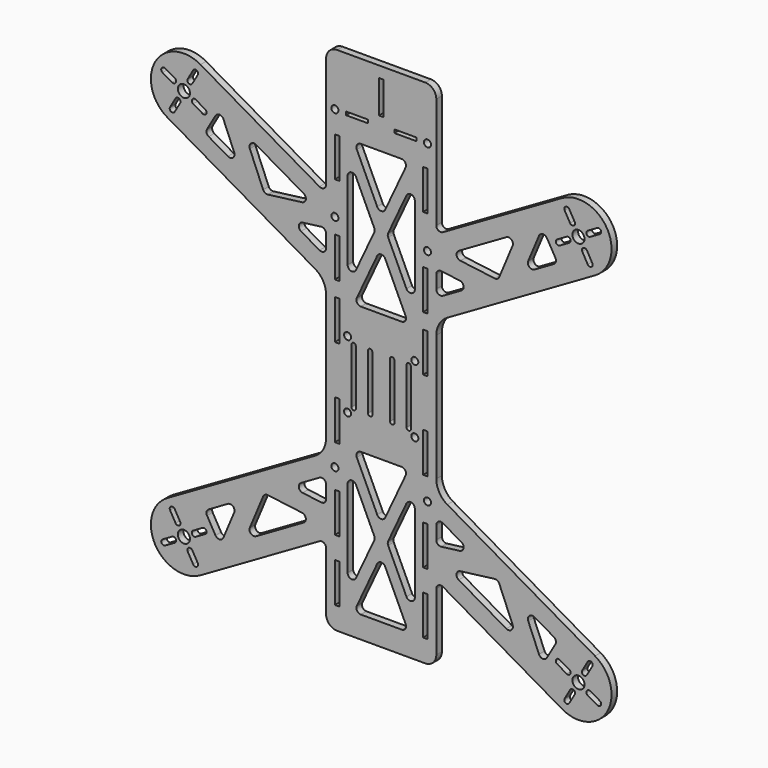
from build123d import *

# Parameters (mm, degrees)
F0_R     = 2.75
F0_W     = 2
F0_H     = 18
F0_R_2   = 1.6
F0_W_2   = 10
F0_H_2   = 1.5
F0_H_3   = 15
F1_DEPTH = 3.175


# Not quite as in the source:
# - ends of sketch curves that miss each other by under 0.0002 mm in the source are joined


with BuildPart() as f1:
    # F0 (on Front) → F1 (new body)
    with BuildSketch(Plane.XZ):
        with BuildLine():
            ThreePointArc((-25, 60.545517), (-26.0000001748, 58.8134660915), (-28.0000003497, 58.8134663943))
            Line((-28.0000003497, 58.8134663943), (-82, 89.990381))
            ThreePointArc((-82, 89.990381), (-102.4903810426, 84.5000000246), (-97.0000000246, 64.0096189574))
            Line((-97.0000000246, 64.0096189574), (-30, 25.327151))
            ThreePointArc((-30, 25.327151), (-26.3397459574, 21.6668969918), (-25, 16.666897))
            Line((-25, 16.666897), (-25, -40.666897))
            ThreePointArc((-25, -40.666897), (-26.3397459574, -45.6668969918), (-29.9999999836, -49.3271510284))
            Line((-29.9999999836, -49.3271510284), (-97, -88.009619))
            ThreePointArc((-97, -88.009619), (-102.4903810426, -108.5000000246), (-81.9999999754, -113.9903810426))
            Line((-81.9999999754, -113.9903810426), (-28, -82.813467))
            ThreePointArc((-28, -82.813467), (-26.0000001748, -82.8134660915), (-25, -84.545517))
            Line((-25, -84.545517), (-25, -111))
            ThreePointArc((-25, -111), (-23.5355339059, -114.5355339059), (-20, -116))
            Line((-20, -116), (20, -116))
            ThreePointArc((20, -116), (23.5355339059, -114.5355339059), (25, -111))
            Line((25, -111), (25, -84.545517))
            ThreePointArc((25, -84.545517), (26.0000001748, -82.8134660915), (28.0000003497, -82.8134663943))
            Line((28.0000003497, -82.8134663943), (82, -113.990381))
            ThreePointArc((82, -113.990381), (102.4903810426, -108.5000000246), (97.0000000246, -88.0096189574))
            Line((97.0000000246, -88.0096189574), (30, -49.327151))
            ThreePointArc((30, -49.327151), (26.3397459574, -45.6668969918), (25, -40.666897))
            Line((25, -40.666897), (25, 16.666897))
            ThreePointArc((25, 16.666897), (26.3397459574, 21.6668969918), (29.9999999836, 25.3271510284))
            Line((29.9999999836, 25.3271510284), (97, 64.009619))
            ThreePointArc((97, 64.009619), (102.4903810426, 84.5000000246), (81.9999999754, 89.9903810426))
            Line((81.9999999754, 89.9903810426), (28, 58.813467))
            ThreePointArc((28, 58.813467), (26.0000001748, 58.8134660915), (25, 60.545517))
            Line((25, 60.545517), (25, 111))
            ThreePointArc((25, 111), (23.5355339059, 114.5355339059), (20, 116))
            Line((20, 116), (-20, 116))
            ThreePointArc((-20, 116), (-23.5355339059, 114.5355339059), (-25, 111))
            Line((-25, 111), (-25, 60.545517))
        make_face()
        with BuildLine():
            ThreePointArc((-94.8631402098, -102.7107696366), (-93.2239096366, -103.1499997902), (-93.6631397902, -104.7892303634))
            Line((-93.6631397902, -104.7892303634), (-97.993267, -107.28923))
            ThreePointArc((-97.993267, -107.28923), (-99.6324973634, -106.8500002098), (-99.1932672098, -105.2107696366))
            Line((-99.1932672098, -105.2107696366), (-94.8631402098, -102.7107696366))
        make_face(mode=Mode.SUBTRACT)
        with BuildLine():
            ThreePointArc((-87.7892303634, -106.3631402098), (-87.3500002098, -104.7239096366), (-85.7107696366, -105.1631397902))
            Line((-85.7107696366, -105.1631397902), (-83.21077, -109.493267))
            ThreePointArc((-83.21077, -109.493267), (-83.6499997902, -111.1324973634), (-85.2892303634, -110.6932672098))
            Line((-85.2892303634, -110.6932672098), (-87.7892303634, -106.3631402098))
        make_face(mode=Mode.SUBTRACT)
        with BuildLine():
            ThreePointArc((-91.2107696366, -95.6368597902), (-91.6499997902, -97.2760903634), (-93.2892303634, -96.8368602098))
            Line((-93.2892303634, -96.8368602098), (-95.78923, -92.506733))
            ThreePointArc((-95.78923, -92.506733), (-95.3500002098, -90.8675026366), (-93.7107696366, -91.3067327902))
            Line((-93.7107696366, -91.3067327902), (-91.2107696366, -95.6368597902))
        make_face(mode=Mode.SUBTRACT)
        with Locations((-89.5, -101)):
            Circle(F0_R, mode=Mode.SUBTRACT)
        with BuildLine():
            ThreePointArc((-84.1368597902, -99.2892303634), (-85.7760903634, -98.8500002098), (-85.3368602098, -97.2107696366))
            Line((-85.3368602098, -97.2107696366), (-81.006733, -94.71077))
            ThreePointArc((-81.006733, -94.71077), (-79.3675026366, -95.1499997902), (-79.8067327902, -96.7892303634))
            Line((-79.8067327902, -96.7892303634), (-84.1368597902, -99.2892303634))
        make_face(mode=Mode.SUBTRACT)
        with BuildLine():
            ThreePointArc((-79.0096188557, -89.1698729167), (-79.2094196277, -87.6522348169), (-78.2775679167, -86.4378221443))
            Line((-78.2775679167, -86.4378221443), (-69.539197, -81.392721))
            ThreePointArc((-69.539197, -81.392721), (-67.2175903894, -81.6236537612), (-66.6944217571, -83.8973031017))
            Line((-66.6944217571, -83.8973031017), (-71.592563, -95.593878))
            ThreePointArc((-71.592563, -95.593878), (-73.3104041105, -96.8173148824), (-75.1693888557, -95.8213469167))
            Line((-75.1693888557, -95.8213469167), (-79.0096188557, -89.1698729167))
        make_face(mode=Mode.SUBTRACT)
        with Locations((-20, -97)):
            Rectangle(F0_W, F0_H, mode=Mode.SUBTRACT)
        with BuildLine():
            ThreePointArc((-9.257183, -106), (-10.9439659593, -105.0745991105), (-11.0697984676, -103.1547632482))
            Line((-11.0697984676, -103.1547632482), (-1.812616, -83.302671))
            ThreePointArc((-1.812616, -83.302671), (0, -82.147907), (1.8126158507, -83.3026710696))
            Line((1.8126158507, -83.3026710696), (11.069799, -103.154763))
            ThreePointArc((11.069799, -103.154763), (10.9439659593, -105.0745991105), (9.257183, -106))
            Line((9.257183, -106), (-9.257183, -106))
        make_face(mode=Mode.SUBTRACT)
        with BuildLine():
            ThreePointArc((-56.7584760833, -90.1795758557), (-59.0800826106, -89.9486432388), (-59.6032512429, -87.6749938983))
            Line((-59.6032512429, -87.6749938983), (-53.553313, -73.227971))
            ThreePointArc((-53.553313, -73.227971), (-52.708538039, -72.268451215), (-51.4551820272, -72.0166142131))
            Line((-51.4551820272, -72.0166142131), (-35.918724, -74.000726))
            ThreePointArc((-35.918724, -74.000726), (-34.2112701558, -75.5906282709), (-35.1720800833, -77.7166648557))
            Line((-35.1720800833, -77.7166648557), (-56.7584760833, -90.1795758557))
        make_face(mode=Mode.SUBTRACT)
        with BuildLine():
            ThreePointArc((-35.6447150984, -65.9707467709), (-37.3521688567, -64.380844667), (-36.3913589167, -62.2548081443))
            Line((-36.3913589167, -62.2548081443), (-28, -57.410055))
            ThreePointArc((-28, -57.410055), (-26.0000001748, -57.4100540915), (-25, -59.142105))
            Line((-25, -59.142105), (-25, -65.058492))
            ThreePointArc((-25, -65.058492), (-25.6783933917, -66.5596102408), (-27.2533559728, -67.0423797869))
            Line((-27.2533559728, -67.0423797869), (-35.6447150984, -65.9707467709))
        make_face(mode=Mode.SUBTRACT)
        with BuildLine():
            ThreePointArc((-11.4373841493, -92.1120459304), (-13.6828789084, -93.2194020851), (-15.25, -91.26681))
            Line((-15.25, -91.26681), (-15.25, -55.73319))
            ThreePointArc((-15.25, -55.73319), (-13.6828789084, -53.7805979149), (-11.4373841493, -54.8879540696))
            Line((-11.4373841493, -54.8879540696), (-3.152585, -72.654763))
            ThreePointArc((-3.152585, -72.654763), (-2.965201, -73.5), (-3.1525855324, -74.3452367518))
            Line((-3.1525855324, -74.3452367518), (-11.4373841493, -92.1120459304))
        make_face(mode=Mode.SUBTRACT)
        with Locations((-20, -69)):
            Rectangle(F0_W, F0_H, mode=Mode.SUBTRACT)
        with Locations((-21, -51)):
            Circle(F0_R_2, mode=Mode.SUBTRACT)
        with BuildLine():
            ThreePointArc((1.8126158507, -63.6973289304), (0, -64.852093), (-1.8126158507, -63.6973289304))
            Line((-1.8126158507, -63.6973289304), (-11.069799, -43.845237))
            ThreePointArc((-11.069799, -43.845237), (-10.9439659593, -41.9254008895), (-9.257183, -41))
            Line((-9.257183, -41), (9.257183, -41))
            ThreePointArc((9.257183, -41), (10.9439659593, -41.9254008895), (11.0697984676, -43.8452367518))
            Line((11.0697984676, -43.8452367518), (1.8126158507, -63.6973289304))
        make_face(mode=Mode.SUBTRACT)
        with Locations((-20, -32)):
            Rectangle(F0_W, F0_H, mode=Mode.SUBTRACT)
        with Locations((-15.25, -27.25)):
            Circle(F0_R_2, mode=Mode.SUBTRACT)
        with BuildLine():
            Line((-13.5, -24.5), (-13.5, 0.5))
            ThreePointArc((-13.5, 0.5), (-12.5, 1.5), (-11.5, 0.5))
            Line((-11.5, 0.5), (-11.5, -24.5))
            ThreePointArc((-11.5, -24.5), (-12.5, -25.5), (-13.5, -24.5))
        make_face(mode=Mode.SUBTRACT)
        with BuildLine():
            Line((-6, -24.5), (-6, 0.5))
            ThreePointArc((-6, 0.5), (-5, 1.5), (-4, 0.5))
            Line((-4, 0.5), (-4, -24.5))
            ThreePointArc((-4, -24.5), (-5, -25.5), (-6, -24.5))
        make_face(mode=Mode.SUBTRACT)
        with Locations((20, -97)):
            Rectangle(F0_W, F0_H, mode=Mode.SUBTRACT)
        with BuildLine():
            ThreePointArc((15.25, -91.26681), (13.6828789084, -93.2194020851), (11.4373841493, -92.1120459304))
            Line((11.4373841493, -92.1120459304), (3.152585, -74.345237))
            ThreePointArc((3.152585, -74.345237), (2.965201, -73.5), (3.1525855324, -72.6547632482))
            Line((3.1525855324, -72.6547632482), (11.437384, -54.887954))
            ThreePointArc((11.437384, -54.887954), (13.6828789084, -53.7805979149), (15.25, -55.73319))
            Line((15.25, -55.73319), (15.25, -91.26681))
        make_face(mode=Mode.SUBTRACT)
        with Locations((20, -69)):
            Rectangle(F0_W, F0_H, mode=Mode.SUBTRACT)
        with BuildLine():
            ThreePointArc((59.6032512429, -87.6749938983), (59.0800826106, -89.9486432388), (56.7584760833, -90.1795758557))
            Line((56.7584760833, -90.1795758557), (35.17208, -77.716665))
            ThreePointArc((35.17208, -77.716665), (34.2112701558, -75.5906282709), (35.9187240272, -74.0007262131))
            Line((35.9187240272, -74.0007262131), (51.455182, -72.016614))
            ThreePointArc((51.455182, -72.016614), (52.708538039, -72.268451215), (53.5533132429, -73.2279708983))
            Line((53.5533132429, -73.2279708983), (59.6032512429, -87.6749938983))
        make_face(mode=Mode.SUBTRACT)
        with BuildLine():
            ThreePointArc((36.3913589167, -62.2548081443), (37.3521688567, -64.380844667), (35.6447150984, -65.9707467709))
            Line((35.6447150984, -65.9707467709), (27.253356, -67.04238))
            ThreePointArc((27.253356, -67.04238), (25.6783933917, -66.5596102408), (25, -65.058492))
            Line((25, -65.058492), (25, -59.142105))
            ThreePointArc((25, -59.142105), (26.0000001748, -57.4100540915), (28.0000003497, -57.4100543943))
            Line((28.0000003497, -57.4100543943), (36.3913589167, -62.2548081443))
        make_face(mode=Mode.SUBTRACT)
        with BuildLine():
            ThreePointArc((78.2775679167, -86.4378221443), (79.2094196277, -87.6522348169), (79.0096188557, -89.1698729167))
            Line((79.0096188557, -89.1698729167), (75.169389, -95.821347))
            ThreePointArc((75.169389, -95.821347), (73.3104041105, -96.8173148824), (71.5925627571, -95.5938781017))
            Line((71.5925627571, -95.5938781017), (66.694422, -83.897303))
            ThreePointArc((66.694422, -83.897303), (67.2175903894, -81.6236537612), (69.5391969167, -81.3927211443))
            Line((69.5391969167, -81.3927211443), (78.2775679167, -86.4378221443))
        make_face(mode=Mode.SUBTRACT)
        with BuildLine():
            Line((83.21077, -109.493267), (85.71077, -105.16314))
            ThreePointArc((85.71077, -105.16314), (87.3500002098, -104.7239096366), (87.7892303634, -106.3631402098))
            Line((87.7892303634, -106.3631402098), (85.28923, -110.693267))
            ThreePointArc((85.28923, -110.693267), (83.6499997902, -111.1324973634), (83.21077, -109.493267))
        make_face(mode=Mode.SUBTRACT)
        with BuildLine():
            Line((97.993267, -107.28923), (93.66314, -104.78923))
            ThreePointArc((93.66314, -104.78923), (93.2239096366, -103.1499997902), (94.8631402098, -102.7107696366))
            Line((94.8631402098, -102.7107696366), (99.193267, -105.21077))
            ThreePointArc((99.193267, -105.21077), (99.6324973634, -106.8500002098), (97.993267, -107.28923))
        make_face(mode=Mode.SUBTRACT)
        with BuildLine():
            Line((81.006733, -94.71077), (85.33686, -97.21077))
            ThreePointArc((85.33686, -97.21077), (85.7760903634, -98.8500002098), (84.1368597902, -99.2892303634))
            Line((84.1368597902, -99.2892303634), (79.806733, -96.78923))
            ThreePointArc((79.806733, -96.78923), (79.3675026366, -95.1499997902), (81.006733, -94.71077))
        make_face(mode=Mode.SUBTRACT)
        with Locations((89.5, -101)):
            Circle(F0_R, mode=Mode.SUBTRACT)
        with BuildLine():
            Line((95.78923, -92.506733), (93.28923, -96.83686))
            ThreePointArc((93.28923, -96.83686), (91.6499997902, -97.2760903634), (91.2107696366, -95.6368597902))
            Line((91.2107696366, -95.6368597902), (93.71077, -91.306733))
            ThreePointArc((93.71077, -91.306733), (95.3500002098, -90.8675026366), (95.78923, -92.506733))
        make_face(mode=Mode.SUBTRACT)
        with Locations((21, -51)):
            Circle(F0_R_2, mode=Mode.SUBTRACT)
        with Locations((20, -32)):
            Rectangle(F0_W, F0_H, mode=Mode.SUBTRACT)
        with Locations((15.25, -27.25)):
            Circle(F0_R_2, mode=Mode.SUBTRACT)
        with BuildLine():
            ThreePointArc((4, 0.5), (5, 1.5), (6, 0.5))
            Line((6, 0.5), (6, -24.5))
            ThreePointArc((6, -24.5), (5, -25.5), (4, -24.5))
            Line((4, -24.5), (4, 0.5))
        make_face(mode=Mode.SUBTRACT)
        with BuildLine():
            ThreePointArc((11.5, 0.5), (12.5, 1.5), (13.5, 0.5))
            Line((13.5, 0.5), (13.5, -24.5))
            ThreePointArc((13.5, -24.5), (12.5, -25.5), (11.5, -24.5))
            Line((11.5, -24.5), (11.5, 0.5))
        make_face(mode=Mode.SUBTRACT)
        with Locations((-15.25, 3.25)):
            Circle(F0_R_2, mode=Mode.SUBTRACT)
        with Locations((-20, 8)):
            Rectangle(F0_W, F0_H, mode=Mode.SUBTRACT)
        with BuildLine():
            ThreePointArc((-9.257183, 17), (-10.9439659593, 17.9254008895), (-11.0697984676, 19.8452367518))
            Line((-11.0697984676, 19.8452367518), (-1.812616, 39.697329))
            ThreePointArc((-1.812616, 39.697329), (0, 40.852093), (1.8126158507, 39.6973289304))
            Line((1.8126158507, 39.6973289304), (11.069799, 19.845237))
            ThreePointArc((11.069799, 19.845237), (10.9439659593, 17.9254008895), (9.257183, 17))
            Line((9.257183, 17), (-9.257183, 17))
        make_face(mode=Mode.SUBTRACT)
        with BuildLine():
            ThreePointArc((-27.2533559728, 43.0423797869), (-25.6783933917, 42.5596102408), (-25, 41.058492))
            Line((-25, 41.058492), (-25, 35.142105))
            ThreePointArc((-25, 35.142105), (-26.0000001748, 33.4100540915), (-28.0000003497, 33.4100543943))
            Line((-28.0000003497, 33.4100543943), (-36.391359, 38.254808))
            ThreePointArc((-36.391359, 38.254808), (-37.3521688567, 40.380844667), (-35.6447150984, 41.9707467709))
            Line((-35.6447150984, 41.9707467709), (-27.2533559728, 43.0423797869))
        make_face(mode=Mode.SUBTRACT)
        with BuildLine():
            ThreePointArc((-35.1720800833, 53.7166648557), (-34.2112701558, 51.5906282709), (-35.9187240272, 50.0007262131))
            Line((-35.9187240272, 50.0007262131), (-51.455182, 48.016614))
            ThreePointArc((-51.455182, 48.016614), (-52.708538039, 48.268451215), (-53.5533132429, 49.2279708983))
            Line((-53.5533132429, 49.2279708983), (-59.603251, 63.674994))
            ThreePointArc((-59.603251, 63.674994), (-59.0800826106, 65.9486432388), (-56.7584760833, 66.1795758557))
            Line((-56.7584760833, 66.1795758557), (-35.1720800833, 53.7166648557))
        make_face(mode=Mode.SUBTRACT)
        with Locations((-20, 33)):
            Rectangle(F0_W, F0_H, mode=Mode.SUBTRACT)
        with Locations((-21, 49)):
            Circle(F0_R_2, mode=Mode.SUBTRACT)
        with BuildLine():
            ThreePointArc((-15.25, 67.26681), (-13.6828789084, 69.2194020851), (-11.4373841493, 68.1120459304))
            Line((-11.4373841493, 68.1120459304), (-3.152585, 50.345237))
            ThreePointArc((-3.152585, 50.345237), (-2.965201, 49.5), (-3.1525855324, 48.6547632482))
            Line((-3.1525855324, 48.6547632482), (-11.437384, 30.887954))
            ThreePointArc((-11.437384, 30.887954), (-13.6828789084, 29.7805979149), (-15.25, 31.73319))
            Line((-15.25, 31.73319), (-15.25, 67.26681))
        make_face(mode=Mode.SUBTRACT)
        with BuildLine():
            ThreePointArc((-93.7107696366, 67.3067327902), (-95.3500002098, 66.8675026366), (-95.7892303634, 68.5067332098))
            Line((-95.7892303634, 68.5067332098), (-93.28923, 72.83686))
            ThreePointArc((-93.28923, 72.83686), (-91.6499997902, 73.2760903634), (-91.2107696366, 71.6368597902))
            Line((-91.2107696366, 71.6368597902), (-93.7107696366, 67.3067327902))
        make_face(mode=Mode.SUBTRACT)
        with BuildLine():
            ThreePointArc((-99.1932672098, 81.2107696366), (-99.6324973634, 82.8500002098), (-97.9932667902, 83.2892303634))
            Line((-97.9932667902, 83.2892303634), (-93.66314, 80.78923))
            ThreePointArc((-93.66314, 80.78923), (-93.2239096366, 79.1499997902), (-94.8631402098, 78.7107696366))
            Line((-94.8631402098, 78.7107696366), (-99.1932672098, 81.2107696366))
        make_face(mode=Mode.SUBTRACT)
        with Locations((-89.5, 77)):
            Circle(F0_R, mode=Mode.SUBTRACT)
        with BuildLine():
            ThreePointArc((-79.8067327902, 72.7892303634), (-79.3675026366, 71.1499997902), (-81.0067332098, 70.7107696366))
            Line((-81.0067332098, 70.7107696366), (-85.33686, 73.21077))
            ThreePointArc((-85.33686, 73.21077), (-85.7760903634, 74.8500002098), (-84.1368597902, 75.2892303634))
            Line((-84.1368597902, 75.2892303634), (-79.8067327902, 72.7892303634))
        make_face(mode=Mode.SUBTRACT)
        with BuildLine():
            ThreePointArc((-85.2892303634, 86.6932672098), (-83.6499997902, 87.1324973634), (-83.2107696366, 85.4932667902))
            Line((-83.2107696366, 85.4932667902), (-85.71077, 81.16314))
            ThreePointArc((-85.71077, 81.16314), (-87.3500002098, 80.7239096366), (-87.7892303634, 82.3631402098))
            Line((-87.7892303634, 82.3631402098), (-85.2892303634, 86.6932672098))
        make_face(mode=Mode.SUBTRACT)
        with BuildLine():
            ThreePointArc((-75.1693888557, 71.8213469167), (-73.3104041105, 72.8173148824), (-71.5925627571, 71.5938781017))
            Line((-71.5925627571, 71.5938781017), (-66.694422, 59.897303))
            ThreePointArc((-66.694422, 59.897303), (-67.2175903894, 57.6236537612), (-69.5391969167, 57.3927211443))
            Line((-69.5391969167, 57.3927211443), (-78.277568, 62.437822))
            ThreePointArc((-78.277568, 62.437822), (-79.2094196277, 63.6522348169), (-79.0096188557, 65.1698729167))
            Line((-79.0096188557, 65.1698729167), (-75.1693888557, 71.8213469167))
        make_face(mode=Mode.SUBTRACT)
        with Locations((-20, 73)):
            Rectangle(F0_W, F0_H, mode=Mode.SUBTRACT)
        with Locations((-21, 92)):
            Circle(F0_R_2, mode=Mode.SUBTRACT)
        with Locations((-11, 92)):
            Rectangle(F0_W_2, F0_H_2, mode=Mode.SUBTRACT)
        with Locations((15.25, 3.25)):
            Circle(F0_R_2, mode=Mode.SUBTRACT)
        with Locations((20, 8)):
            Rectangle(F0_W, F0_H, mode=Mode.SUBTRACT)
        with Locations((20, 33)):
            Rectangle(F0_W, F0_H, mode=Mode.SUBTRACT)
        with BuildLine():
            Line((15.25, 67.26681), (15.25, 31.73319))
            ThreePointArc((15.25, 31.73319), (13.6828789084, 29.7805979149), (11.4373841493, 30.8879540696))
            Line((11.4373841493, 30.8879540696), (3.152585, 48.654763))
            ThreePointArc((3.152585, 48.654763), (2.965201, 49.5), (3.1525855324, 50.3452367518))
            Line((3.1525855324, 50.3452367518), (11.437384, 68.112046))
            ThreePointArc((11.437384, 68.112046), (13.6828789084, 69.2194020851), (15.25, 67.26681))
        make_face(mode=Mode.SUBTRACT)
        with Locations((21, 49)):
            Circle(F0_R_2, mode=Mode.SUBTRACT)
        with BuildLine():
            ThreePointArc((25, 41.058492), (25.6783933917, 42.5596102408), (27.2533559728, 43.0423797869))
            Line((27.2533559728, 43.0423797869), (35.644715, 41.970746))
            ThreePointArc((35.644715, 41.970746), (37.3521688567, 40.380844667), (36.3913589167, 38.2548081443))
            Line((36.3913589167, 38.2548081443), (28, 33.410055))
            ThreePointArc((28, 33.410055), (26.0000001748, 33.4100540915), (25, 35.142105))
            Line((25, 35.142105), (25, 41.058492))
        make_face(mode=Mode.SUBTRACT)
        with BuildLine():
            ThreePointArc((56.7584760833, 66.1795758557), (59.0800826106, 65.9486432388), (59.6032512429, 63.6749938983))
            Line((59.6032512429, 63.6749938983), (53.553313, 49.227971))
            ThreePointArc((53.553313, 49.227971), (52.708538039, 48.268451215), (51.4551820272, 48.0166142131))
            Line((51.4551820272, 48.0166142131), (35.918724, 50.000726))
            ThreePointArc((35.918724, 50.000726), (34.2112701558, 51.5906282709), (35.1720800833, 53.7166648557))
            Line((35.1720800833, 53.7166648557), (56.7584760833, 66.1795758557))
        make_face(mode=Mode.SUBTRACT)
        with BuildLine():
            ThreePointArc((1.8126158507, 59.3026710696), (0, 58.147907), (-1.8126158507, 59.3026710696))
            Line((-1.8126158507, 59.3026710696), (-11.069799, 79.154763))
            ThreePointArc((-11.069799, 79.154763), (-10.9439659593, 81.0745991105), (-9.257183, 82))
            Line((-9.257183, 82), (9.257183, 82))
            ThreePointArc((9.257183, 82), (10.9439659593, 81.0745991105), (11.0697984676, 79.1547632482))
            Line((11.0697984676, 79.1547632482), (1.8126158507, 59.3026710696))
        make_face(mode=Mode.SUBTRACT)
        with Locations((20, 73)):
            Rectangle(F0_W, F0_H, mode=Mode.SUBTRACT)
        with Locations((11, 92)):
            Rectangle(F0_W_2, F0_H_2, mode=Mode.SUBTRACT)
        with Locations((21, 92)):
            Circle(F0_R_2, mode=Mode.SUBTRACT)
        with Locations((0, 103.5)):
            Rectangle(F0_W, F0_H_3, mode=Mode.SUBTRACT)
        with BuildLine():
            ThreePointArc((71.5925627571, 71.5938781017), (73.3104041105, 72.8173148824), (75.1693888557, 71.8213469167))
            Line((75.1693888557, 71.8213469167), (79.009619, 65.169873))
            ThreePointArc((79.009619, 65.169873), (79.2094196277, 63.6522348169), (78.2775679167, 62.4378221443))
            Line((78.2775679167, 62.4378221443), (69.539197, 57.392721))
            ThreePointArc((69.539197, 57.392721), (67.2175903894, 57.6236537612), (66.6944217571, 59.8973031017))
            Line((66.6944217571, 59.8973031017), (71.5925627571, 71.5938781017))
        make_face(mode=Mode.SUBTRACT)
        with BuildLine():
            ThreePointArc((95.7892303634, 68.5067332098), (95.3500002098, 66.8675026366), (93.7107696366, 67.3067327902))
            Line((93.7107696366, 67.3067327902), (91.21077, 71.63686))
            ThreePointArc((91.21077, 71.63686), (91.6499997902, 73.2760903634), (93.2892303634, 72.8368602098))
            Line((93.2892303634, 72.8368602098), (95.7892303634, 68.5067332098))
        make_face(mode=Mode.SUBTRACT)
        with BuildLine():
            ThreePointArc((81.0067332098, 70.7107696366), (79.3675026366, 71.1499997902), (79.8067327902, 72.7892303634))
            Line((79.8067327902, 72.7892303634), (84.13686, 75.28923))
            ThreePointArc((84.13686, 75.28923), (85.7760903634, 74.8500002098), (85.3368602098, 73.2107696366))
            Line((85.3368602098, 73.2107696366), (81.0067332098, 70.7107696366))
        make_face(mode=Mode.SUBTRACT)
        with Locations((89.5, 77)):
            Circle(F0_R, mode=Mode.SUBTRACT)
        with BuildLine():
            ThreePointArc((83.2107696366, 85.4932667902), (83.6499997902, 87.1324973634), (85.2892303634, 86.6932672098))
            Line((85.2892303634, 86.6932672098), (87.78923, 82.36314))
            ThreePointArc((87.78923, 82.36314), (87.3500002098, 80.7239096366), (85.7107696366, 81.1631397902))
            Line((85.7107696366, 81.1631397902), (83.2107696366, 85.4932667902))
        make_face(mode=Mode.SUBTRACT)
        with BuildLine():
            ThreePointArc((97.9932667902, 83.2892303634), (99.6324973634, 82.8500002098), (99.1932672098, 81.2107696366))
            Line((99.1932672098, 81.2107696366), (94.86314, 78.71077))
            ThreePointArc((94.86314, 78.71077), (93.2239096366, 79.1499997902), (93.6631397902, 80.7892303634))
            Line((93.6631397902, 80.7892303634), (97.9932667902, 83.2892303634))
        make_face(mode=Mode.SUBTRACT)
    extrude(amount=F1_DEPTH)


solid = f1.part
